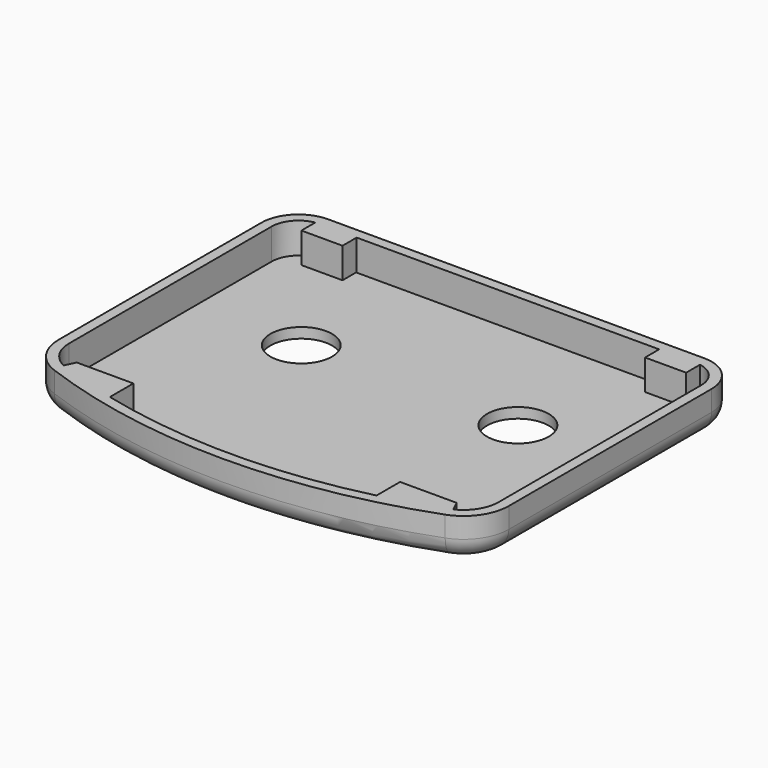
from build123d import *

# Parameters (mm, degrees)
F1_DEPTH = 12.7
F2_T     = -3.175
F3_R     = 6.35
F5_W     = 12.7
F5_H     = 6.35
F6_DEPTH = 9.398
F7_R     = 9.525
F8_DEPTH = 25.4


# Not quite as in the source:
# - a feature names something its author has since deleted; it is built from what else it names


with BuildPart() as f1:
    # F0 (on Top) → F1 (new body)
    with BuildSketch(Plane.XY):
        with BuildLine():
            Line((58.0965084505, 62.5356453779), (-58.0965084505, 62.5356453779))
            ThreePointArc((-58.0965084505, 62.5356453779), (-66.1787389595, 59.1878758868), (-69.5265084505, 51.1056453779))
            Line((-69.5265084505, 51.1056453779), (-69.5265084505, -27.1992570698))
            ThreePointArc((-69.5265084505, -27.1992570698), (-67.0115325937, -35.1957139026), (-60.3721316603, -40.3130159932))
            ThreePointArc((-60.3721316603, -40.3130159932), (0, -51.0474727306), (60.3721316603, -40.3130159932))
            ThreePointArc((60.3721316603, -40.3130159932), (67.0115325937, -35.1957139026), (69.5265084505, -27.1992570698))
            Line((69.5265084505, -27.1992570698), (69.5265084505, 51.1056453779))
            ThreePointArc((69.5265084505, 51.1056453779), (66.1787389595, 59.1878758868), (58.0965084505, 62.5356453779))
        make_face()
    extrude(amount=F1_DEPTH)

    # F2
    f2_openings = [f1.faces().sort_by_distance(p)[0] for p in [
        (0, 7.919531, 12.7),
    ]]
    offset(amount=F2_T, openings=f2_openings)

    # F3
    f3_edges = [f1.edges().sort_by_distance(p)[0] for p in [
        (69.526508, 11.953194, 0),
        (66.178739, 59.187876, 0),
        (0, 62.535645, 0),
        (-66.178739, 59.187876, 0),
        (-69.526508, 11.953194, 0),
        (-67.011533, -35.195714, 0),
        (0, -51.047473, 0),
        (67.011533, -35.195714, 0),
    ]]
    fillet(f3_edges, radius=F3_R)

    # F5 (on offset) → F6 (join)
    with BuildSketch(Plane.XY.offset(12.7)):
        with Locations((-53.0805146158, 57.0815077901)):
            Rectangle(F5_W, F5_H)
        with Locations((53.0805146158, 57.0815077901)):
            Rectangle(F5_W, F5_H)
        Polygon((-41.1868803203, -33.773638308), (-58.6946308613, -33.773638308), (-60.6418885291, -37.9110425711), (-53.9016760886, -40.266495198), (-41.1868803203, -43.3214269578), align=None)
        Polygon((60.6418885291, -37.9110425711), (58.6946308613, -33.773638308), (41.1868803203, -33.773638308), (41.1868803203, -43.3214269578), (53.9016760886, -40.266495198), align=None)
    extrude(amount=-F6_DEPTH)

    # F7 (on face) → F8 (cut)
    with BuildSketch(Plane.XY.offset(3.175)):
        with Locations((-33.4585084505, 21.3863216341)):
            Circle(F7_R)
        with Locations((33.4585084505, 21.3863216341)):
            Circle(F7_R)
    extrude(amount=-F8_DEPTH, mode=Mode.SUBTRACT)


solid = f1.part
